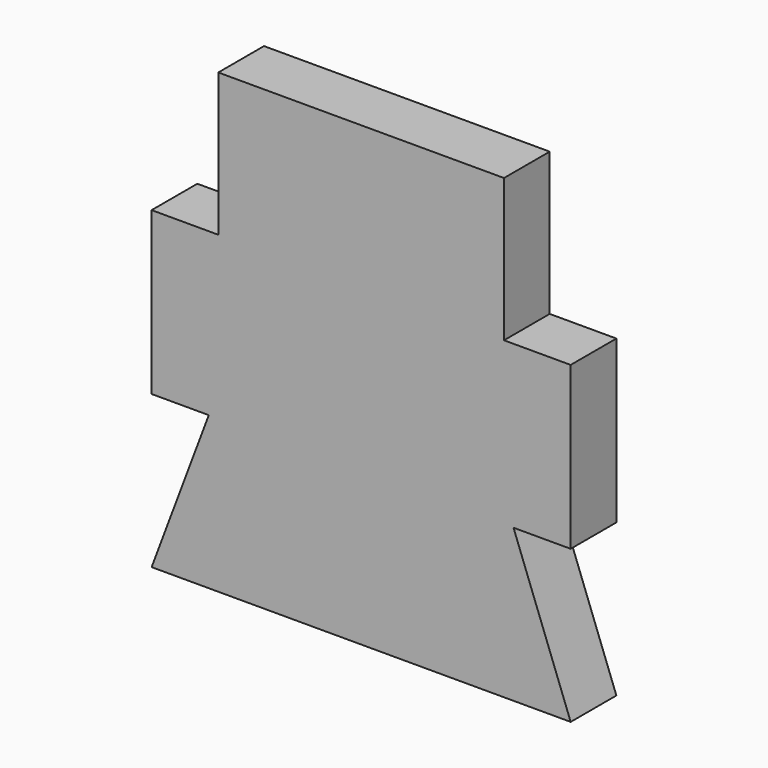
from build123d import *

# Parameters (mm, degrees)
F0_W     = 139.7
F0_H     = 152.4
F1_DEPTH = 19.05
F2_W     = 22.225
F2_H     = 47.625
F3_DEPTH = 19.051
F6_DEPTH = 19.051


# Not quite as in the source:
# - a length typed as a fraction of an inch, garbled in the dataset ("3 / 203.2 mm" for 3/8 in), is restored
# - a pattern or mirror of a feature is missing from the dataset's text; its kind, count and spacing are read off the source's solid


with BuildPart() as f1:
    # F0 (on Front) → F1 (new body)
    with BuildSketch(Plane.XZ):
        with Locations((69.85, 76.2)):
            Rectangle(F0_W, F0_H)
    extrude(amount=F1_DEPTH)

    # F2 (on face) → F3 (cut, through all)
    with BuildSketch(Plane.XZ.offset(19.05)):
        with Locations((11.1125, 128.5875)):
            Rectangle(F2_W, F2_H)
    f3 = extrude(amount=-F3_DEPTH, mode=Mode.SUBTRACT)

    # F3_copies: F3 across plane
    add(f3.mirror(Plane(origin=(69.85, 0, 0), x_dir=(0, 0, 1), z_dir=(1, 0, 0))), mode=Mode.SUBTRACT)

    # F5 (on face) → F6 (cut, through all)
    with BuildSketch(Plane.XZ.offset(19.05)):
        Polygon((0, 50.8), (0, 0), (19.05, 50.8), align=None)
    f6 = extrude(amount=-F6_DEPTH, mode=Mode.SUBTRACT)

    # F6_copies: F6 across plane
    add(f6.mirror(Plane(origin=(69.85, 0, 0), x_dir=(0, 0, 1), z_dir=(1, 0, 0))), mode=Mode.SUBTRACT)


solid = f1.part
